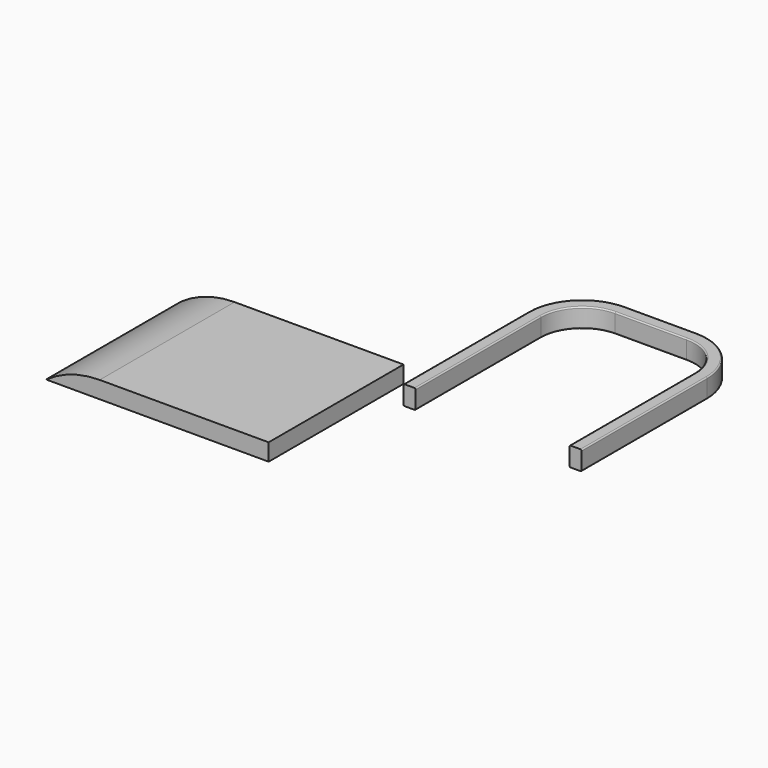
from build123d import *

# Parameters (mm, degrees)
F2_W        = 26.4934301376
F2_H        = 20.0631171465
F3_DEPTH    = 2.032
F4_T1_DEPTH = 51.9725717919


# Not quite as in the source:
# - a fillet or chamfer that OpenCascade refuses, or shapes differently, is made with other operations: its cross-section is extruded or revolved along the edge and cut away or added


with BuildPart() as f3:
    # F2 (on Top) → F3 (new body)
    with BuildSketch(Plane.XY):
        with Locations((-13.2467150688, -10.0315585732)):
            Rectangle(F2_W, F2_H)
    extrude(amount=F3_DEPTH)

    # F4: fillet of radius 11.0377844072 on 1 edges, made by hand

    # F4_s2 → F4_t1 (cut)
    with BuildSketch(Plane.XZ.offset(-15.9547273227)):
        with BuildLine():
            ThreePointArc((-26.4934301376, 0), (-23.4603283864, 1.5117388593), (-20.1115392085, 2.032))
            Line((-20.1115392085, 2.032), (-26.4934301376, 2.032))
            Line((-26.4934301376, 2.032), (-26.4934301376, 0))
        make_face()
    extrude(amount=F4_T1_DEPTH, mode=Mode.SUBTRACT)


with BuildPart() as f5:
    # F5: sweep along a path in F0
    with BuildLine(Plane.XY) as f5_path:
        Line((0, 0), (0, 18.6531258911))
        ThreePointArc((0, 18.6531258911), (1.8598719395, 23.1432539516), (6.35, 25.0031258911))
        Line((6.35, 25.0031258911), (14.8563547224, 25.0031258911))
        ThreePointArc((14.8563547224, 25.0031258911), (19.3464827829, 23.1432539516), (21.2063547224, 18.6531258911))
        Line((21.2063547224, 18.6531258911), (21.2063547224, 0))
    # F1 (on Front) → F5 (sweep)
    with BuildSketch(Plane.XZ):
        with BuildLine():
            Line((1.30386401, 0), (0.1471562355, 0))
            ThreePointArc((0.1471562355, 0), (0.0431010635, -0.0431010635), (0, -0.1471562355))
            Line((0, -0.1471562355), (0, -2.1458242045))
            ThreePointArc((0, -2.1458242045), (0.0431010635, -2.2498793765), (0.1471562355, -2.29298044))
            Line((0.1471562355, -2.29298044), (1.30386401, -2.29298044))
            ThreePointArc((1.30386401, -2.29298044), (1.407919182, -2.2498793765), (1.4510202454, -2.1458242045))
            Line((1.4510202454, -2.1458242045), (1.4510202454, -0.1471562355))
            ThreePointArc((1.4510202454, -0.1471562355), (1.407919182, -0.0431010635), (1.30386401, 0))
        make_face()
    sweep(path=f5_path.line)


solid = Compound([f3.part, f5.part])
